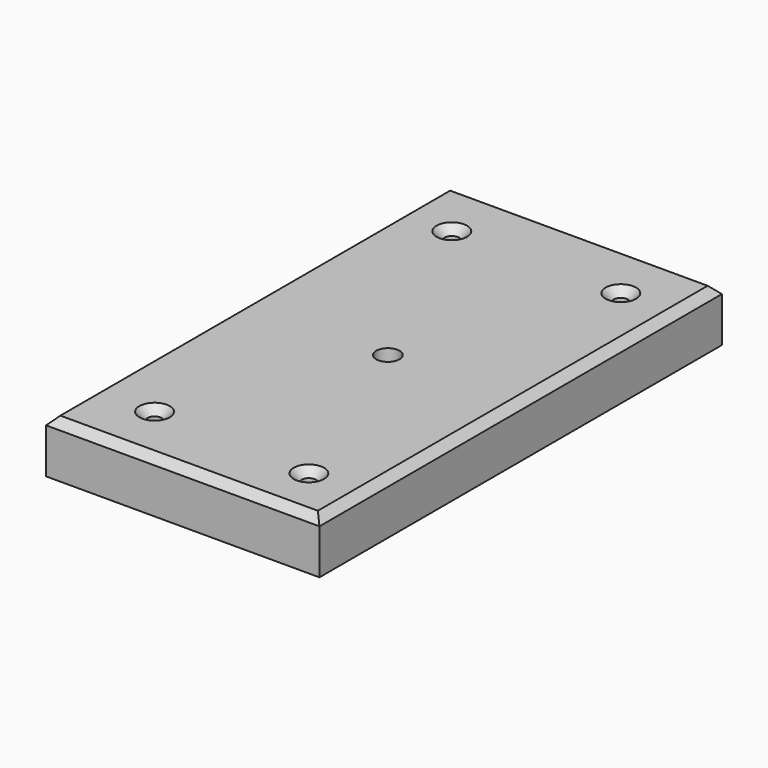
from build123d import *

# Parameters (mm, degrees)
F0_W     = 103.4416258335
F0_H     = 190.3689950705
F1_DEPTH = 20
F3_D     = 5.5
F4_SIZE  = 3
F6_D     = 8.8


# Not quite as in the source:
# - a feature names something its author has since deleted; it is built from what else it names


with BuildPart() as f1:
    # F0 (on Top) → F1 (new body)
    with BuildSketch(Plane.XY):
        with Locations((-51.7208129168, 95.1844975352)):
            Rectangle(F0_W, F0_H)
    extrude(amount=F1_DEPTH)

    # F3 (through all)
    with Locations(Plane.XY.offset(20)):
        with Locations((-20, 20), (-83.82, 167.386), (-20.066, 167.64), (-80.264, 22.352)):
            Hole(F3_D / 2)

    # F4
    f4_edges = [f1.edges().sort_by_distance(p)[0] for p in [
        (-51.720813, 0, 20),
        (-103.441626, 95.184498, 20),
        (0, 95.184498, 20),
        (-51.720813, 190.368995, 20),
        (-83.014, 22.352, 20),
        (-22.75, 20, 20),
        (-86.57, 167.386, 20),
        (-22.816, 167.64, 20),
    ]]
    chamfer(f4_edges, length=F4_SIZE)

    # F6 (through all)
    with Locations(Plane.XY.offset(20)):
        with Locations((-49.0952916443, 93.7389880419)):
            Hole(F6_D / 2)


solid = f1.part
